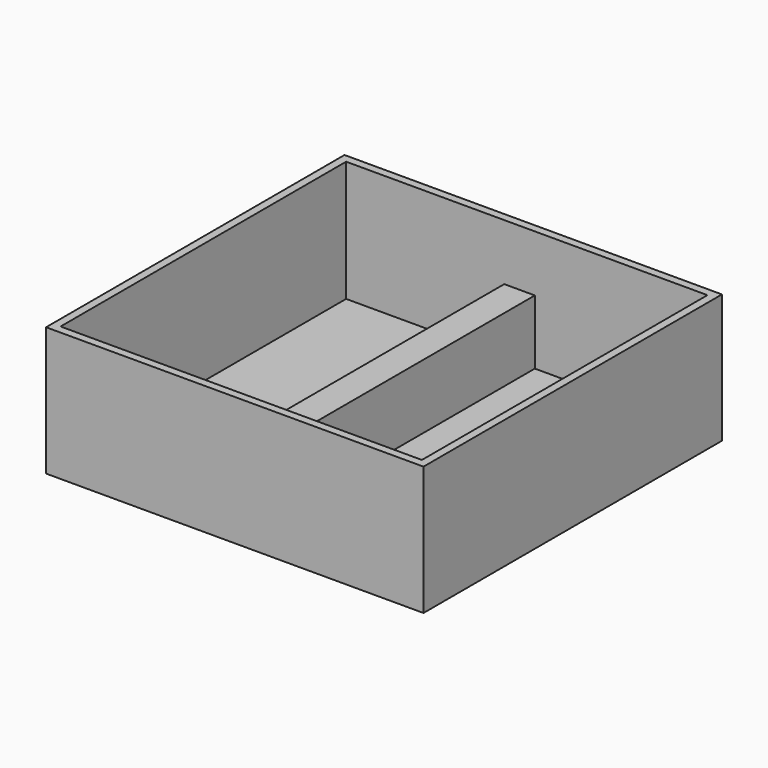
from build123d import *

# Parameters (mm, degrees)
F0_W     = 148.7955749035
F0_H     = 147.0687389374
F1_DEPTH = 50.8
F3_START = -25.4
F2_W     = 5.715
F2_H     = 140.7187389374
F3_DEPTH = 38.1
F4_T     = -3.175


# Not quite as in the source:
# - a shell that OpenCascade refuses in one call is made with other operations: the cavity is built on its own and cut out


with BuildPart() as f1:
    # F0 (on Top) → F1 (new body)
    with BuildSketch(Plane.XY):
        with Locations((0.9957179427, -1.8707364798)):
            Rectangle(F0_W, F0_H)
    extrude(amount=-F1_DEPTH)

    # F2 (on face) → F3 (cut)
    with BuildSketch(Plane.XY.offset(F3_START)):
        with Locations((-1.8617820573, -1.8707364798)):
            Rectangle(F2_W, F2_H)
    extrude(amount=-F3_DEPTH, mode=Mode.SUBTRACT)

    # F4: a shell. OpenCascade refuses it in one call, so the cavity is built on its own and cut out:
    # the body offset inwards by the wall thickness, plus a prism from it out through each open face.
    f4_core = offset(f1.part, amount=F4_T, kind=Kind.INTERSECTION, mode=Mode.PRIVATE)
    f4_exits = [f4_core.faces().sort_by_distance(p)[0] for p in [
        (0.995718, -1.870736, -3.175),
    ]]
    add(f4_core, mode=Mode.SUBTRACT)
    extrude(f4_exits, amount=-F4_T, mode=Mode.SUBTRACT)


solid = f1.part
